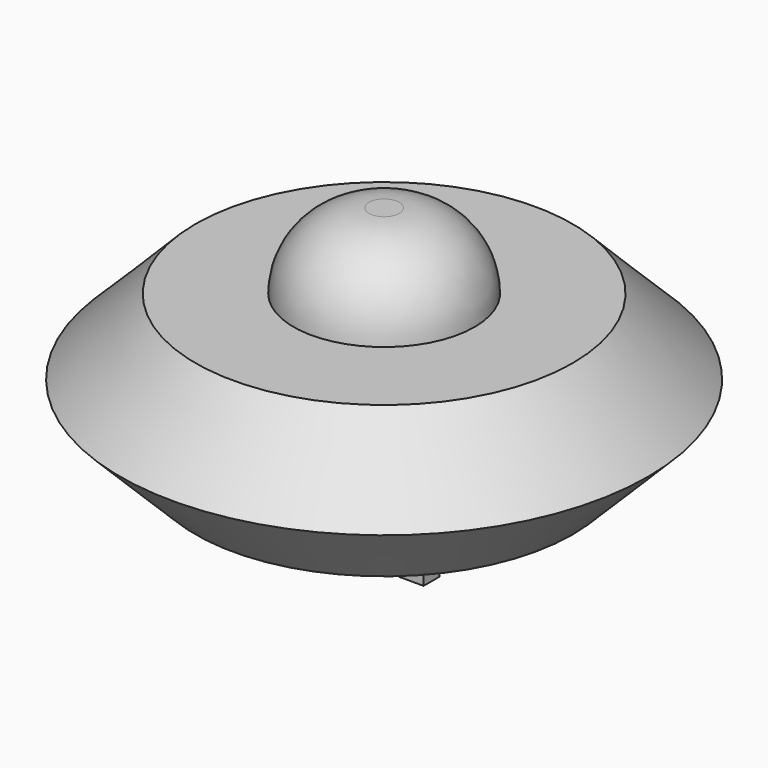
from build123d import *

# Parameters (mm, degrees)
F0_R     = 88.9
F1_DEPTH = 50.8
F2_SIZE  = 25.4
F3_SIZE  = 25.39999
F4_R     = 30.4888877606
F5_DEPTH = 25.4
F6_R     = 25.39999
F7_W     = 8.3943400532
F7_H     = 6.7154671997
F7_W_2   = 8.0585591495
F7_W_3   = 7.0512406528
F7_H_2   = 7.0512406528
F7_H_3   = 7.722787559
F8_DEPTH = 12.7


# Not quite as in the source:
# - a fillet or chamfer is up to 0.001 mm smaller than in the source, because OpenCascade refuses the exact size


with BuildPart() as f1:
    # F0 (on Top) → F1 (new body)
    with BuildSketch(Plane.XY):
        Circle(F0_R)
    extrude(amount=F1_DEPTH)

    # F2
    f2_edges = [f1.edges().sort_by_distance(p)[0] for p in [
        (-88.9, 0, 50.8),
    ]]
    chamfer(f2_edges, length=F2_SIZE)

    # F3 (size 25.4 in the source; OpenCascade refuses exactly that, so slightly less here)
    f3_edges = [f1.edges().sort_by_distance(p)[0] for p in [
        (-88.9, 0, 0),
    ]]
    chamfer(f3_edges, length=F3_SIZE)

    # F4 (on face) → F5 (join)
    with BuildSketch(Plane.XY.offset(50.8)):
        Circle(F4_R)
    extrude(amount=F5_DEPTH)

    # F6 (radius 25.4 in the source; OpenCascade refuses exactly that, so slightly less here)
    f6_edges = [f1.edges().sort_by_distance(p)[0] for p in [
        (-30.488888, 0, 76.2),
    ]]
    fillet(f6_edges, radius=F6_R)

    # F7 (on face) → F8 (join)
    with BuildSketch(Plane(origin=(0, 0, 0), x_dir=(1, 0, 0), z_dir=(0, 0, -1))):
        with Locations((31.7305838689, 24.918817915)):
            Rectangle(F7_W, F7_H)
        with Locations((-29.8838298768, 24.918817915)):
            Rectangle(F7_W_2, F7_H)
        with Locations((-29.3801706284, -27.6297163218)):
            Rectangle(F7_W_3, F7_H_2)
        with Locations((31.7305838689, -27.2939428687)):
            Rectangle(F7_W, F7_H_3)
    extrude(amount=F8_DEPTH)


solid = f1.part
